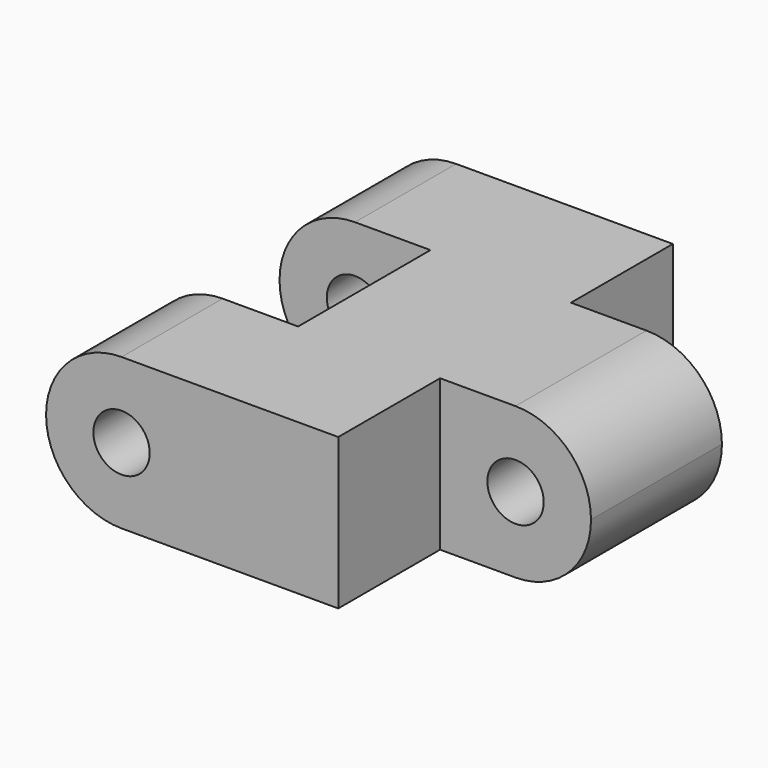
from build123d import *

# Parameters (mm, degrees)
F1_DEPTH = 8.3
F2_R     = 1.55
F3_DEPTH = 23.001
F4_R     = 1.55
F5_DEPTH = 16.001
F6_R     = 4.14999


# Not quite as in the source:
# - a fillet or chamfer is up to 0.001 mm smaller than in the source, because OpenCascade refuses the exact size


with BuildPart() as f1:
    # F0 (on Top) → F1 (new body)
    with BuildSketch(Plane.XY):
        Polygon((-57.5197213515, -7.7541078215), (-65.8197213515, -7.7541078215), (-65.8197213515, -14.7041078215), (-49.7500874824, -14.7041078215), (-49.7500874824, -7.7041078215), (-41.4500874824, -7.7041078215), (-41.4500874824, 1.2958921785), (-49.7500874824, 1.2958921785), (-49.7500874824, 8.2958921785), (-65.8197213515, 8.2958921785), (-65.8197213515, 1.3458921785), (-57.5197213515, 1.3458921785), align=None)
    extrude(amount=F1_DEPTH)

    # F2 (on face) → F3 (cut, through all)
    with BuildSketch(Plane.XZ.offset(14.7041078215)):
        with Locations((-61.6697213515, 4.15)):
            Circle(F2_R)
    extrude(amount=-F3_DEPTH, mode=Mode.SUBTRACT)

    # F4 (on face) → F5 (cut, through all)
    with BuildSketch(Plane.XZ.offset(7.7041078215)):
        with Locations((-45.6000874824, 4.15)):
            Circle(F4_R)
    extrude(amount=-F5_DEPTH, mode=Mode.SUBTRACT)

    # F6 (radius 4.15 in the source; OpenCascade refuses exactly that, so slightly less here)
    f6_edges = [f1.edges().sort_by_distance(p)[0] for p in [
        (-65.819721, 4.820892, 8.3),
        (-65.819721, 4.820892, 0),
        (-65.819721, -11.229108, 0),
        (-65.819721, -11.229108, 8.3),
        (-41.450087, -3.204108, 0),
        (-41.450087, -3.204108, 8.3),
    ]]
    fillet(f6_edges, radius=F6_R)


solid = f1.part
